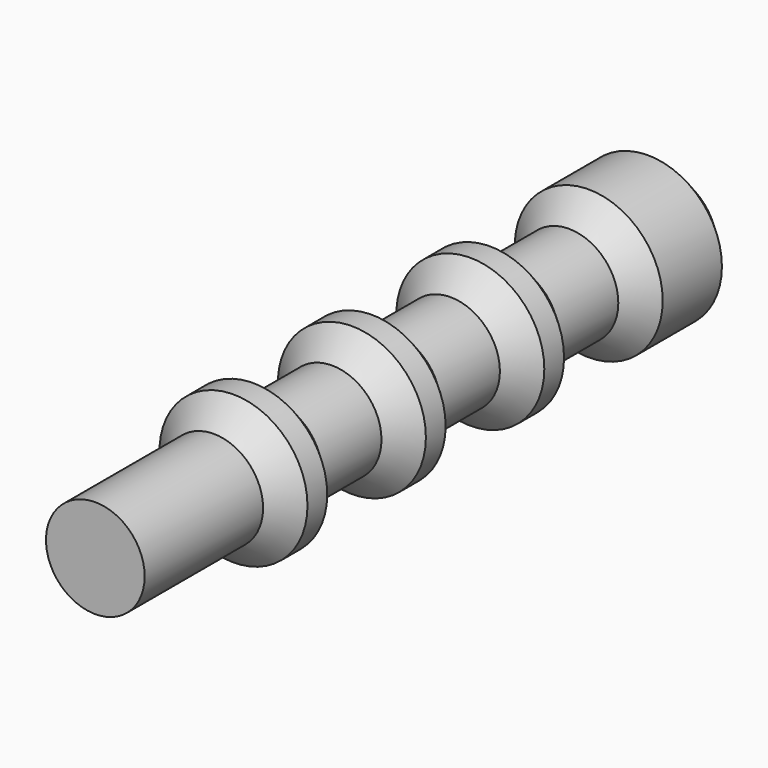
from build123d import *

# Parameters (mm, degrees)
F2_SIZE = 4.99999


# Not quite as in the source:
# - a fillet or chamfer is up to 0.001 mm smaller than in the source, because OpenCascade refuses the exact size
# - a feature names something its author has since deleted; it is built from what else it names


with BuildPart() as f1:
    # F0 (on Top) → F1 (revolve)
    with BuildSketch(Plane.XY):
        Polygon((0, 145), (0, 0), (10, 0), (10, 30), (15, 30), (15, 45), (10, 45), (10, 60), (15, 60), (15, 75), (10, 75), (10, 90), (15, 90), (15, 105), (10, 105), (10, 120), (15, 120), (15, 145), align=None)
    revolve(axis=Axis((0, 72.5, 0), (0, 1, 0)))

    # F2 (size 5 in the source; OpenCascade refuses exactly that, so slightly less here)
    f2_edges = [f1.edges().sort_by_distance(p)[0] for p in [
        (-15, 105, 0),
        (-15, 90, 0),
        (-15, 75, 0),
        (-15, 60, 0),
        (-15, 45, 0),
        (-15, 30, 0),
        (-15, 120, 0),
        (-15, 145, 0),
    ]]
    chamfer(f2_edges, length=F2_SIZE)


solid = f1.part
